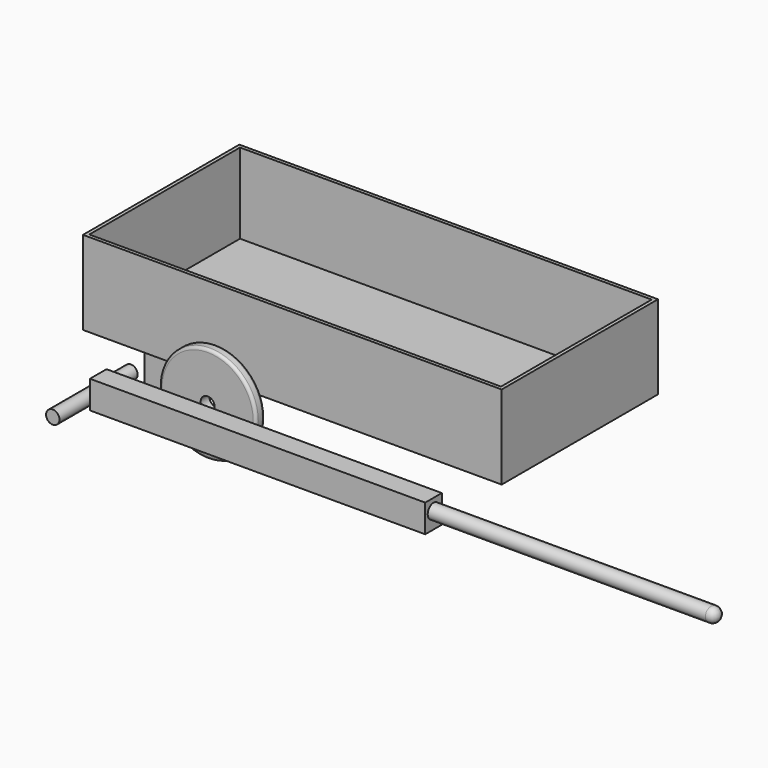
from build123d import *

# Parameters (mm, degrees)
F0_W      = 75.3477662802
F0_H      = 19.5513167419
F3_R      = 5.08
F4_R      = 12.192
F5_DEPTH  = 177.8
F6_W      = 762
F6_H      = 355.6
F7_DEPTH  = 152.4
F8_T      = -6.35
F9_W      = 76.2
F9_H      = 25.4
F10_DEPTH = 152.4
F11_R     = 15.875
F12_DEPTH = 279.401
F13_W     = 610.290300101
F13_H     = 37.7013385296
F14_DEPTH = 50.8
F15_R     = 13.1863448391
F16_DEPTH = 508


with BuildPart() as f2:
    # F0 (on Top) → F2 (revolve)
    with BuildSketch(Plane.XY):
        with Locations((37.6738831401, 4.5118422713)):
            Rectangle(F0_W, F0_H)
    revolve(axis=Axis((-12.7, 0, 0.664958757), (0, -1, 0)))

    # F3
    f3_edges = [f2.edges().sort_by_distance(p)[0] for p in [
        (-100.747766, 14.287501, 1.329918),
        (-100.747766, -5.263816, 1.329918),
    ]]
    fillet(f3_edges, radius=F3_R)


with BuildPart() as f5:
    # F4 (on Front) → F5 (new body)
    with BuildSketch(Plane.XZ):
        with Locations((-156.5919518471, 3.3260271885)):
            Circle(F4_R)
    extrude(amount=F5_DEPTH)


with BuildPart() as f7:
    # F6 (on Top) → F7 (new body)
    with BuildSketch(Plane.XY):
        with Locations((86.3827507496, 241.3377019644)):
            Rectangle(F6_W, F6_H)
    extrude(amount=F7_DEPTH)

    # F8
    f8_openings = [f7.faces().sort_by_distance(p)[0] for p in [
        (86.382751, 241.337702, 152.4),
    ]]
    offset(amount=F8_T, openings=f8_openings)

    # F9 (on face) → F10 (join)
    with BuildSketch(Plane(origin=(0, 0, 0), x_dir=(1, 0, 0), z_dir=(0, 0, -1))):
        with Locations((-205.7172492504, -152.4377019644)):
            Rectangle(F9_W, F9_H)
        with Locations((-205.7172492504, -330.2377019644)):
            Rectangle(F9_W, F9_H)
    extrude(amount=F10_DEPTH)

    # F11 (on face) → F12 (cut, through all)
    with BuildSketch(Plane.XZ.offset(-139.7377019644)):
        with Locations((-205.7172492504, -112.3936101794)):
            Circle(F11_R)
    extrude(amount=-F12_DEPTH, mode=Mode.SUBTRACT)


with BuildPart() as f14:
    # F13 (on Top) → F14 (new body)
    with BuildSketch(Plane.XY):
        with Locations((172.9780230671, -104.9500331283)):
            Rectangle(F13_W, F13_H)
    extrude(amount=F14_DEPTH)

    # F15 (on face) → F16 (join)
    with BuildSketch(Plane.YZ.offset(478.1231731176)):
        with Locations((-104.9500331283, 29.8119243234)):
            Circle(F15_R)
    extrude(amount=F16_DEPTH)

    # F17 (on face) → F18 (revolve)
    with BuildSketch(Plane.YZ.offset(986.1231731176)):
        with BuildLine():
            ThreePointArc((-91.7636882892, 29.8119243234), (-95.8917593375, 39.3945839828), (-105.6913334808, 42.977415731))
            Line((-105.6913334808, 42.977415731), (-104.4964387545, 16.6333833435))
            ThreePointArc((-104.4964387545, 16.6333833435), (-95.4668653547, 20.6495436725), (-91.7636882892, 29.8119243234))
        make_face()
    revolve(axis=Axis((986.1231731176, -105.0938861176, 29.8053995373), (0, 0.0453107361, -0.9989729412)))


solid = Compound([f2.part, f5.part, f7.part, f14.part])
